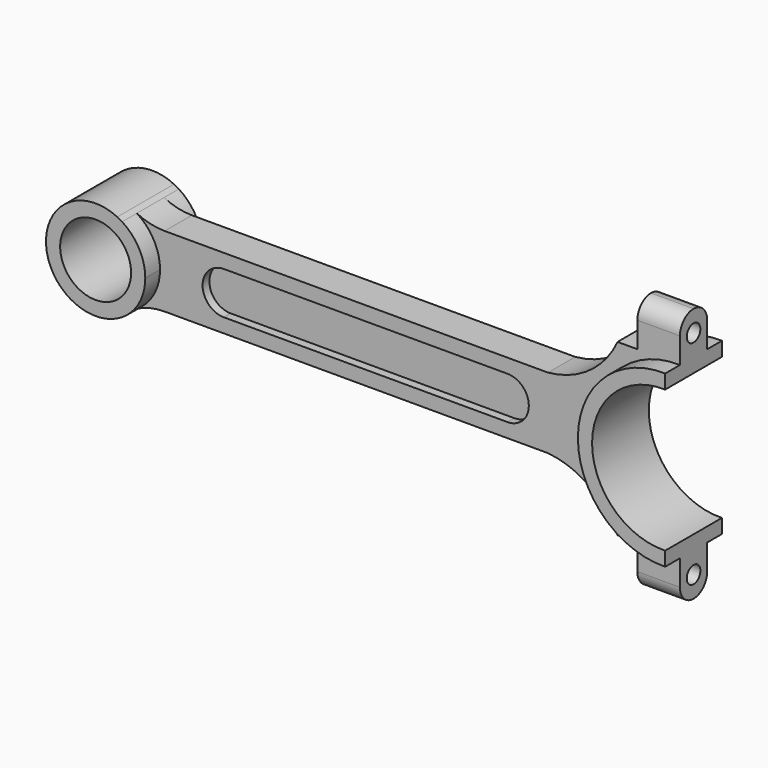
from build123d import *

# Parameters (mm, degrees)
F1_DEPTH  = 12.5
F0_R      = 12.5
F2_DEPTH  = 6
F3_R      = 5.99999
F4_R      = 5.99999
F6_DEPTH  = 3
F8_DEPTH  = 3
F9_R      = 3
F10_DEPTH = 218.2697359261


# Not quite as in the source:
# - a fillet or chamfer is up to 0.001 mm smaller than in the source, because OpenCascade refuses the exact size


with BuildPart() as f1:
    # F0 (on Front) → F1 (new body, symmetric)
    with BuildSketch(Plane.XZ):
        with BuildLine():
            Line((110.9687169417, 24.9881781063), (110.9687169417, 29.9901491338))
            ThreePointArc((110.9687169417, 29.9901491338), (80.1999810155, 2.02996e-05), (110.9686763555, -29.9901501743))
            Line((110.9686763555, -29.9901501743), (110.9686763555, -24.988179355))
            ThreePointArc((110.9686763555, -24.988179355), (85.1999810155, 2.03026e-05), (110.9687169417, 24.9881781063))
        make_face()
    extrude(amount=F1_DEPTH, both=True)



with BuildPart() as f1b:
    # F0 (on Front) → F1, piece 2 (new body, symmetric)
    with BuildSketch(Plane.XZ):
        with BuildLine():
            ThreePointArc((-80.4711318513, 14.8061428082), (-81.3358966232, 15.2609531347), (-82.1796143085, 15.7537117078))
            ThreePointArc((-82.1796143085, 15.7537117078), (-107.3000189845, 0), (-82.1796143085, -15.7537117078))
            ThreePointArc((-82.1796143085, -15.7537117078), (-81.3358966232, -15.2609531347), (-80.4711318513, -14.8061428082))
            ThreePointArc((-80.4711318513, -14.8061428082), (-74.4783753907, -8.455603916), (-72.3000189845, 0))
            ThreePointArc((-72.3000189845, 0), (-74.4783753907, 8.455603916), (-80.4711318513, 14.8061428082))
        make_face()
        with Locations((-89.8000189845, 0)):
            Circle(F0_R, mode=Mode.SUBTRACT)
    extrude(amount=F1_DEPTH, both=True)


with BuildPart() as f1_1:
    add(f1.part)

    add(f1b.part)  # F2 merges F1b
    # F0 (on Front) → F2 (join, symmetric)
    with BuildSketch(Plane.XZ):
        with BuildLine():
            ThreePointArc((-70.6654197961, 12.5), (-75.702042761, 13.0842948024), (-80.4711318513, 14.8061428082))
            ThreePointArc((-80.4711318513, 14.8061428082), (-74.4783753907, 8.455603916), (-72.3000189845, 0))
            ThreePointArc((-72.3000189845, 0), (-74.4783753907, -8.455603916), (-80.4711318513, -14.8061428082))
            ThreePointArc((-80.4711318513, -14.8061428082), (-75.702042761, -13.0842948024), (-70.6654197961, -12.5))
            Line((-70.6654197961, -12.5), (64.4492452955, -12.5))
            ThreePointArc((64.4492452955, -12.5), (79.0647132666, -17.9493308815), (88.9686763555, -30))
            Line((88.9686763555, -30), (95.9686763555, -30))
            Line((95.9686763555, -30), (95.9686763555, -45))
            Line((95.9686763555, -45), (110.9686763555, -45))
            Line((110.9686763555, -45), (110.9686763555, -29.9901501743))
            ThreePointArc((110.9686763555, -29.9901501743), (80.1999810155, 2.02996e-05), (110.9687169417, 29.9901491338))
            Line((110.9687169417, 29.9901491338), (110.9687169417, 45))
            Line((110.9687169417, 45), (95.9687169417, 44.9999957531))
            Line((95.9687169417, 44.9999957531), (95.9687169417, 29.9999957531))
            Line((95.9687169417, 29.9999957531), (88.9687169417, 29.9999957531))
            ThreePointArc((88.9687169417, 29.9999957531), (79.0647357521, 17.9493194217), (64.4492452955, 12.5))
            Line((64.4492452955, 12.5), (-70.6654197961, 12.5))
        make_face()
    extrude(amount=F2_DEPTH, both=True)

    # F3 (radius 6 in the source; OpenCascade refuses exactly that, so slightly less here)
    f3_edges = [f1_1.edges().sort_by_distance(p)[0] for p in [
        (103.468717, -6, 44.999998),
        (103.468717, 6, 44.999998),
    ]]
    fillet(f3_edges, radius=F3_R)

    # F4 (radius 6 in the source; OpenCascade refuses exactly that, so slightly less here)
    f4_edges = [f1_1.edges().sort_by_distance(p)[0] for p in [
        (103.468676, -6, -45),
        (103.468676, 6, -45),
    ]]
    fillet(f4_edges, radius=F4_R)

    # F5 (on face) → F6 (cut)
    with BuildSketch(Plane.XZ.offset(6)):
        with BuildLine():
            Line((50.1999810155, 7.5), (-49.8000189845, 7.5))
            ThreePointArc((-49.8000189845, 7.5), (-57.3000189845, 0), (-49.8000189845, -7.5))
            Line((-49.8000189845, -7.5), (50.1999810155, -7.5))
            ThreePointArc((50.1999810155, -7.5), (57.6999810155, 0), (50.1999810155, 7.5))
        make_face()
    extrude(amount=-F6_DEPTH, mode=Mode.SUBTRACT)

    # F7 (on face) → F8 (cut)
    with BuildSketch(Plane(origin=(0, 6, 0), x_dir=(-1, 0, 0), z_dir=(0, 1, 0))):
        with BuildLine():
            Line((49.8000189845, 7.5), (-50.1999810155, 7.5))
            ThreePointArc((-50.1999810155, 7.5), (-57.6999810155, 0), (-50.1999810155, -7.5))
            Line((-50.1999810155, -7.5), (49.8000189845, -7.5))
            ThreePointArc((49.8000189845, -7.5), (57.3000189845, 0), (49.8000189845, 7.5))
        make_face()
    extrude(amount=-F8_DEPTH, mode=Mode.SUBTRACT)

    # F9 (on face) → F10 (cut, through all)
    with BuildSketch(Plane.YZ.offset(110.9687169417)):
        with Locations((0, 37.5)):
            Circle(F9_R)
        with Locations((0, -37.5)):
            Circle(F9_R)
    extrude(amount=-F10_DEPTH, mode=Mode.SUBTRACT)


solid = f1_1.part
